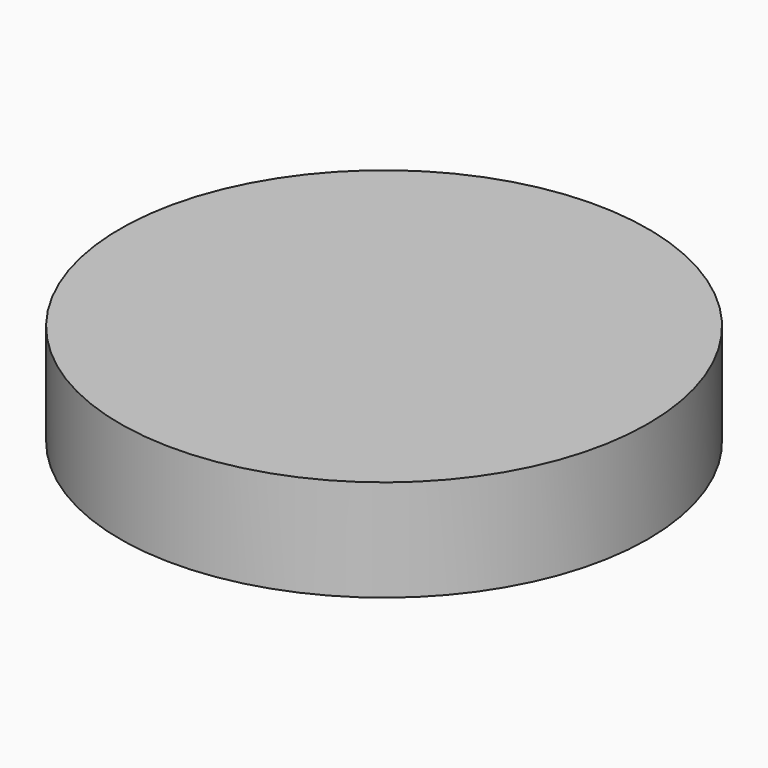
from build123d import *

# Parameters (mm, degrees)
F2_R     = 26
F3_DEPTH = 10


# Not quite as in the source:
# - the program builds the solid bodies; features that only make, move or delete a surface that nothing else refers to are left out


with BuildPart() as f3:
    # F2 (on Top) → F3 (new body)
    with BuildSketch(Plane.XY):
        with Locations((-46.3043488562, 17.1195659786)):
            Circle(F2_R)
    extrude(amount=F3_DEPTH)


solid = f3.part
